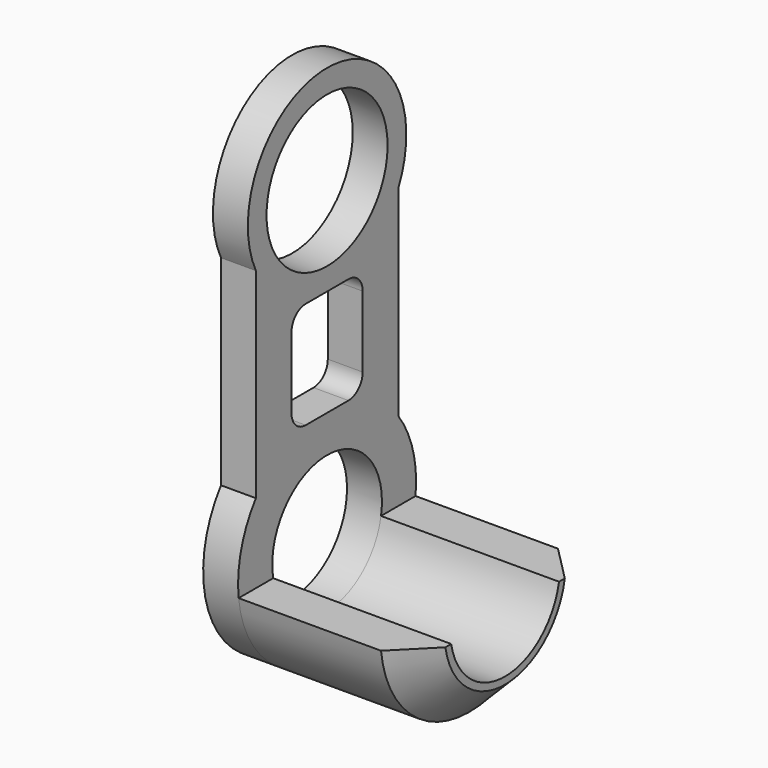
from build123d import *

# Parameters (mm, degrees)
F0_R     = 9.779
F0_W     = 12.7
F0_H     = 15.24
F0_R_2   = 10.795
F1_DEPTH = 4.9800002
F3_DEPTH = 25.4
F4_SIZE  = 5.08
F5_R     = 2.54


# Not quite as in the source:
# - a feature names something its author has since deleted; it is built from what else it names


with BuildPart() as f1:
    # F0 (on Right) → F1 (new body)
    with BuildSketch(Plane.YZ):
        with BuildLine():
            Line((12.7, -34.7691013034), (12.7, -6.1941013034))
            ThreePointArc((12.7, -6.1941013034), (0, 14.12999968), (-12.7, -6.1941013034))
            Line((-12.7, -6.1941013034), (-12.7, -34.7691013034))
            ThreePointArc((-12.7, -34.7691013034), (0, -60.1691013034), (12.7, -34.7691013034))
        make_face()
        with Locations((0, -44.2941013034)):
            Circle(F0_R, mode=Mode.SUBTRACT)
        with Locations((0, -21.59)):
            Rectangle(F0_W, F0_H, mode=Mode.SUBTRACT)
        Circle(F0_R_2, mode=Mode.SUBTRACT)
    extrude(amount=F1_DEPTH)

    # F2 (on face) → F3 (join)
    with BuildSketch(Plane.YZ.offset(4.9800002)):
        with BuildLine():
            ThreePointArc((9.6160052517, -46.0721013034), (0, -54.0731013034), (-9.6160052517, -46.0721013034))
            Line((-9.6160052517, -46.0721013034), (-15.7751177809, -46.0721013034))
            ThreePointArc((-15.7751177809, -46.0721013034), (0, -60.1691013034), (15.7751177809, -46.0721013034))
            Line((15.7751177809, -46.0721013034), (9.6160052517, -46.0721013034))
        make_face()
    extrude(amount=F3_DEPTH)

    # F4
    f4_edges = [f1.edges().sort_by_distance(p)[0] for p in [
        (30.38, 0, -60.169101),
    ]]
    chamfer(f4_edges, length=F4_SIZE)

    # F5
    f5_edges = [f1.edges().sort_by_distance(p)[0] for p in [
        (2.49, 6.35, -13.97),
        (2.49, -6.35, -13.97),
        (2.49, 6.35, -29.21),
        (2.49, -6.35, -29.21),
    ]]
    fillet(f5_edges, radius=F5_R)


solid = f1.part
